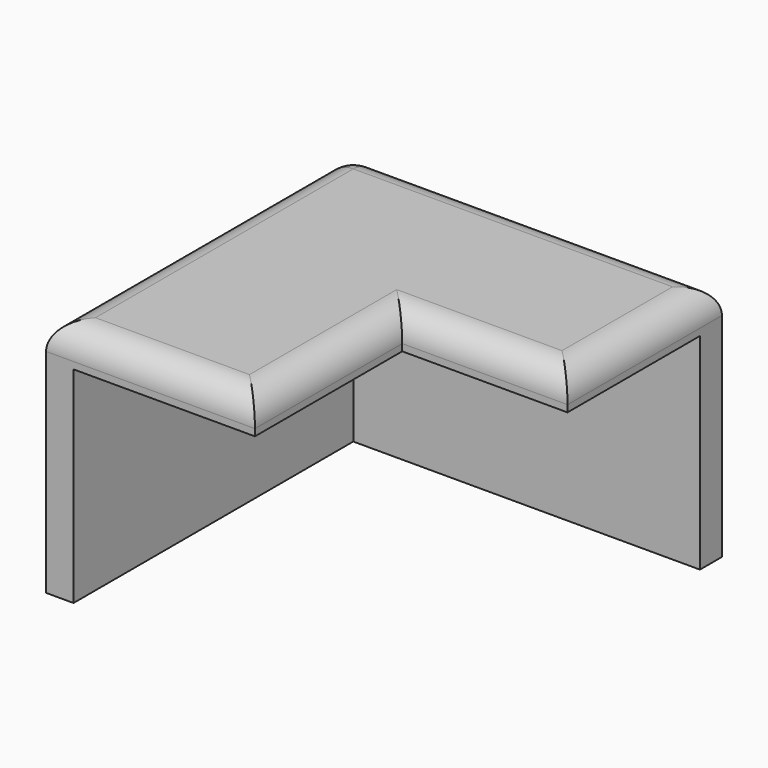
from build123d import *

# Parameters (mm, degrees)
F1_DEPTH    = 6.35
F3_DEPTH    = 38.1
F4_R        = 5.08
F5_T1_DEPTH = 52.07
F5_S5_W     = 5.08
F5_S5_H     = 5.08
F5_T6_DEPTH = 5.08


# Not quite as in the source:
# - a fillet or chamfer that OpenCascade refuses, or shapes differently, is made with other operations: its cross-section is extruded or revolved along the edge and cut away or added


with BuildPart() as f1:
    # F0 (on Top) → F1 (new body)
    with BuildSketch(Plane.XY):
        Polygon((69.2906975746, 0), (0, 0), (0, -69.8406398296), (38.6781543493, -69.8406398296), (38.6781543493, -35.7452183962), (69.2906975746, -35.7452183962), align=None)
    extrude(amount=F1_DEPTH)

    # F2 (on face) → F3 (join)
    with BuildSketch(Plane(origin=(0, 0, 0), x_dir=(1, 0, 0), z_dir=(0, 0, -1))):
        Polygon((5.08, 69.8406398296), (0, 69.8406398296), (0, 0), (69.2906975746, 0), (69.2906975746, 5.08), (5.08, 5.08), align=None)
    extrude(amount=F3_DEPTH)

    # F4
    f4_edges = [f1.edges().sort_by_distance(p)[0] for p in [
        (34.645349, 0, 6.35),
        (0, -34.92032, 6.35),
        (19.339077, -69.84064, 6.35),
        (38.678154, -52.792929, 6.35),
        (53.984426, -35.745218, 6.35),
        (69.290698, -17.872609, 6.35),
    ]]
    fillet(f4_edges, radius=F4_R)

    # F5: fillet of radius 5.08 on 1 edges, made by hand

    # F5_s2 → F5_t1 (cut)
    with BuildSketch(Plane.XY.offset(-50.8)):
        with BuildLine():
            ThreePointArc((5.08, 0), (1.4878975516, -1.4878975516), (0, -5.08))
            Line((0, -5.08), (0, 0))
            Line((0, 0), (5.08, 0))
        make_face()
    extrude(amount=F5_T1_DEPTH, mode=Mode.SUBTRACT)


with BuildPart() as f5_tool4:
    # F5_s5 → F5_t6 (new body)
    with BuildSketch(Plane.XZ.offset(5.08)):
        with Locations((2.54, 3.81)):
            Rectangle(F5_S5_W, F5_S5_H)
    extrude(amount=-F5_T6_DEPTH)

    # F5_s7 → F5_t8 (revolve, cut)
    with BuildSketch(Plane(origin=(5.08, -5.08, 1.27), x_dir=(0.7071067812, 0, -0.7071067812), z_dir=(0.7071067812, 0, 0.7071067812))):
        with BuildLine():
            ThreePointArc((0, -5.08), (5.08, 0), (0, 5.08))
            Line((0, 5.08), (0, -5.08))
        make_face()
    revolve(axis=Axis((5.08, -5.08, 1.27), (0, 1, 0)), mode=Mode.SUBTRACT)


with BuildPart() as f1_1:
    add(f1.part)

    # F5_t3: cut F5_tool4
    add(f5_tool4.part, mode=Mode.SUBTRACT)


solid = f1_1.part
